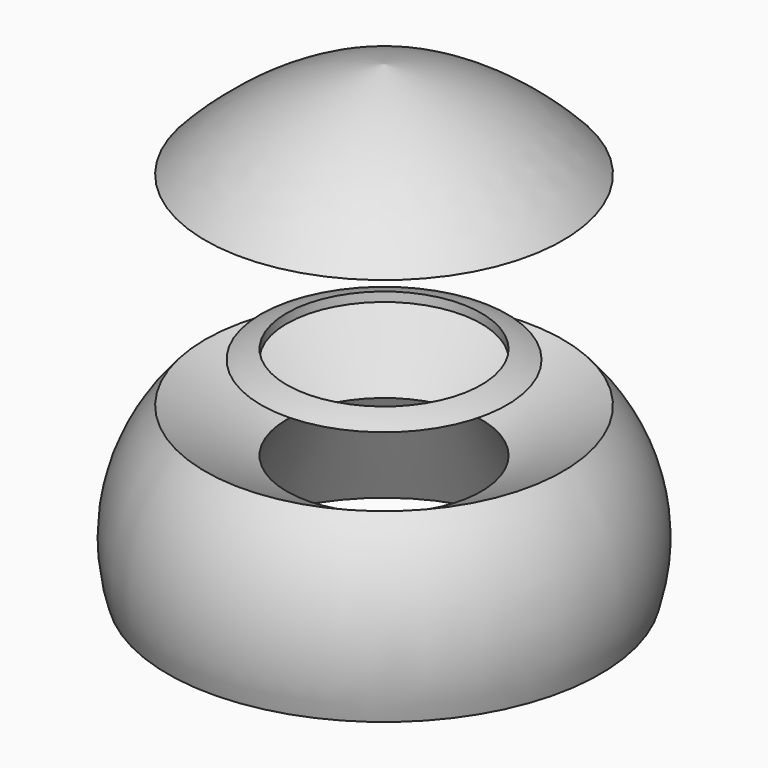
from build123d import *


# Not quite as in the source:
# - the program builds the solid bodies; features that only make, move or delete a surface that nothing else refers to are left out


with BuildPart() as f1:
    # F0 (on Front) → F1 (revolve)
    with BuildSketch(Plane.XZ):
        with BuildLine():
            Line((-31.5, -36.7715619504), (-57.8949571854, -22.5130124036))
            ThreePointArc((-57.8949571854, -22.5130124036), (-71.100893869, -47.8091979463), (-70, -76.3237871839))
            Line((-70, -76.3237871839), (-52.8878243203, -76.3639977286))
            Line((-52.8878243203, -76.3639977286), (-31.5, -36.7715619504))
        make_face()
    revolve(axis=Axis((0, 0, -0.7809376717), (0, 0, -1)))


with BuildPart() as f3:
    # F0 (on Front) → F3 (revolve)
    with BuildSketch(Plane.XZ):
        with BuildLine():
            Line((-31.5, -9.4140620232), (-31.5, -6.4140620232))
            ThreePointArc((-31.5, -6.4140620232), (-35.7282093513, -7.7475284985), (-39.836560988, -9.4140620232))
            Line((-39.836560988, -9.4140620232), (-31.5, -9.4140620232))
        make_face()
    revolve(axis=Axis((0, 0, -0.7809376717), (0, 0, -1)))


with BuildPart() as f3b:
    # F0 (on Front) → F3, piece 2 (revolve)
    with BuildSketch(Plane.XZ):
        with BuildLine():
            Line((-31.5, -36.7715619504), (-57.8949571854, -22.5130124036))
            ThreePointArc((-57.8949571854, -22.5130124036), (-71.100893869, -47.8091979463), (-70, -76.3237871839))
            Line((-70, -76.3237871839), (-52.8878243203, -76.3639977286))
            Line((-52.8878243203, -76.3639977286), (-31.5, -36.7715619504))
        make_face()
    revolve(axis=Axis((0, 0, -0.7809376717), (0, 0, -1)))


with BuildPart() as f3c:
    # F0 (on Front) → F3, piece 3 (revolve)
    with BuildSketch(Plane.XZ):
        with BuildLine():
            Line((0, 46.3521866798), (0, 74.8521866798))
            ThreePointArc((0, 74.8521866798), (-31.3917968408, 63.5946851026), (-57.8949571854, 43.3521866798))
            Line((-57.8949571854, 43.3521866798), (-31.5, 43.3521866798))
            Line((-31.5, 43.3521866798), (-31.5, 46.3521866798))
            Line((-31.5, 46.3521866798), (0, 46.3521866798))
        make_face()
    revolve(axis=Axis((0, 0, -0.7809376717), (0, 0, -1)))


with BuildPart() as f4:
    # F0 (on Front) → F4 (revolve)
    with BuildSketch(Plane.XZ):
        with BuildLine():
            Line((-31.5, -9.4140620232), (-31.5, -6.4140620232))
            ThreePointArc((-31.5, -6.4140620232), (-35.7282093513, -7.7475284985), (-39.836560988, -9.4140620232))
            Line((-39.836560988, -9.4140620232), (-31.5, -9.4140620232))
        make_face()
    revolve(axis=Axis((0, 0, -0.7809376717), (0, 0, -1)))


solid = Compound([f1.part, f3.part, f3b.part, f3c.part, f4.part])
